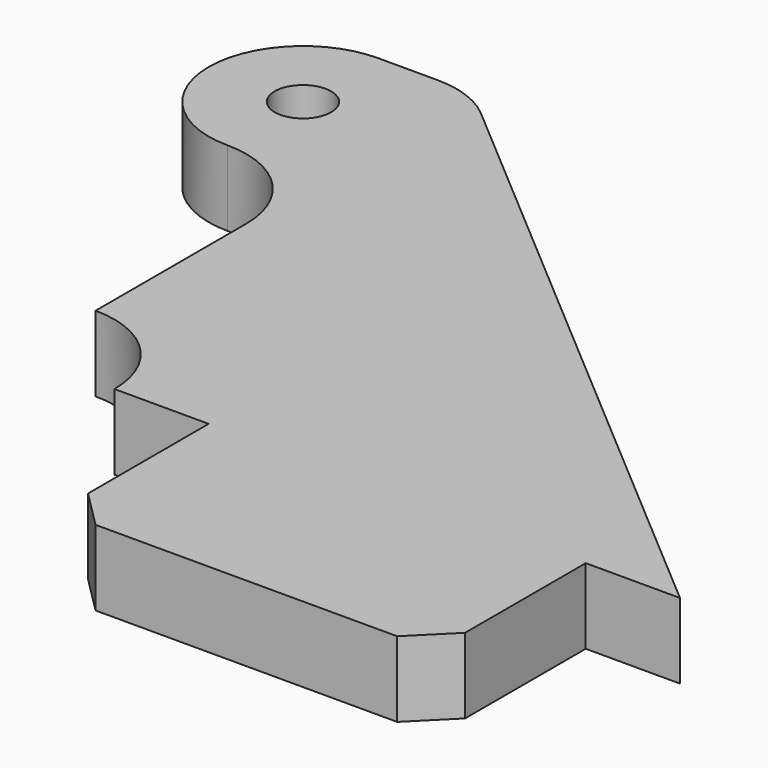
from build123d import *

# Parameters (mm, degrees)
F0_R     = 0.75
F1_DEPTH = 2
F2_R     = 2.49999


# Not quite as in the source:
# - a fillet or chamfer is up to 0.001 mm smaller than in the source, because OpenCascade refuses the exact size


with BuildPart() as f1:
    # F0 (on Top) → F1 (new body)
    with BuildSketch(Plane.XY):
        with BuildLine():
            Line((-10, 0), (-7.5, 0))
            Line((-7.5, 0), (2.5, 0))
            Line((2.5, 0), (5, 0))
            Line((5, 0), (-12.5, 15))
            Line((-12.5, 15), (-17.5, 15))
            Line((-17.5, 15), (-17.5, 10))
            Line((-17.5, 10), (-12.5, 10))
            Line((-12.5, 10), (-12.5, 2.5))
            ThreePointArc((-12.5, 2.5), (-10.732233047, 1.767766953), (-10, 0))
        make_face()
        with Locations((-15, 12.5)):
            Circle(F0_R, mode=Mode.SUBTRACT)
        Polygon((-7.5, -4), (-6.5, -5), (1.5, -5), (2.5, -4), (2.5, 0), (-7.5, 0), align=None)
    extrude(amount=F1_DEPTH)

    # F2 (radius 2.5 in the source; OpenCascade refuses exactly that, so slightly less here)
    f2_edges = [f1.edges().sort_by_distance(p)[0] for p in [
        (-17.5, 15, 1),
        (-17.5, 10, 1),
        (-12.5, 15, 1),
        (-12.5, 10, 1),
    ]]
    fillet(f2_edges, radius=F2_R)


solid = f1.part
